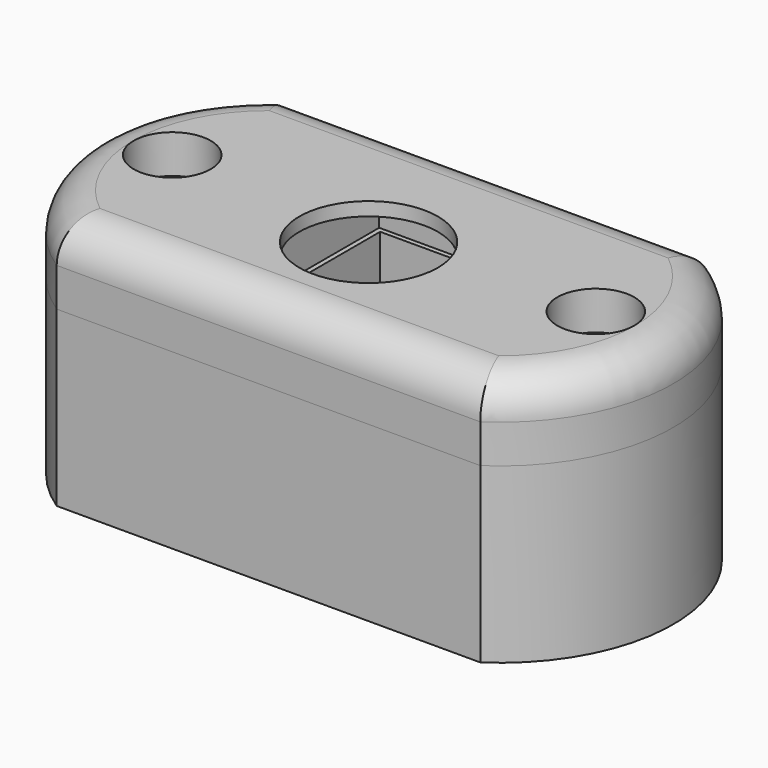
from build123d import *

# Parameters (mm, degrees)
F0_W            = 22
F0_H            = 15
F1_DEPTH        = 9
F2_R            = 1
F2_W            = 10
F2_H            = 12
F3_DEPTH        = 9
F4_W            = 10
F4_H            = 9
F5_DEPTH        = 0.5
F6_W            = 22
F6_H            = 15
F7_DEPTH        = 4
F8_R            = 3.6
F9_DEPTH        = 4
F10_T1_DEPTH    = 32
F10_T4_ANGLE    = 176.5875970816
F10_T6_ANGLE    = 176.5875970816
F11_D           = 2
F11_DEPTH       = 20
F11_CBORE_D     = 4
F11_CBORE_DEPTH = 2
F11_TIP         = 0.600860619
F12_W           = 10.5
F12_H           = 12.5
F13_DEPTH       = 3.3


# Not quite as in the source:
# - a fillet or chamfer that OpenCascade refuses, or shapes differently, is made with other operations: its cross-section is extruded or revolved along the edge and cut away or added


with BuildPart() as f1:
    # F0 (on Top) → F1 (new body)
    with BuildSketch(Plane.XY):
        with Locations((-45, -43.5413755476)):
            Rectangle(F0_W, F0_H)
        with BuildLine():
            ThreePointArc((-34, -51.0413755476), (-29.9749371855, -43.5413755476), (-34, -36.0413755476))
            Line((-34, -36.0413755476), (-34, -51.0413755476))
        make_face()
        with BuildLine():
            Line((-56, -51.0413755476), (-56, -36.0413755476))
            ThreePointArc((-56, -36.0413755476), (-60.0250628145, -43.5413755476), (-56, -51.0413755476))
        make_face()
    extrude(amount=F1_DEPTH)

    # F2 (on face) → F3 (cut)
    with BuildSketch(Plane.XY.offset(9)):
        with Locations((-56, -43.5413755476)):
            Circle(F2_R)
        with Locations((-34, -43.5413755476)):
            Circle(F2_R)
        with Locations((-45, -43.5413755476)):
            Rectangle(F2_W, F2_H)
    extrude(amount=-F3_DEPTH, mode=Mode.SUBTRACT)

    # F4 (on face) → F5 (join)
    with BuildSketch(Plane(origin=(0, 0, 0), x_dir=(1, 0, 0), z_dir=(0, 0, -1))):
        with Locations((-45, 45.0413755476)):
            Rectangle(F4_W, F4_H)
    extrude(amount=-F5_DEPTH)


with BuildPart() as f7:
    # F6 (on face) → F7 (new body)
    with BuildSketch(Plane.XY.offset(9)):
        with Locations((-45, -43.5413755476)):
            Rectangle(F6_W, F6_H)
        with BuildLine():
            ThreePointArc((-34, -51.0413755476), (-29.9749371855, -43.5413755476), (-34, -36.0413755476))
            Line((-34, -36.0413755476), (-34, -51.0413755476))
        make_face()
        with BuildLine():
            Line((-56, -51.0413755476), (-56, -36.0413755476))
            ThreePointArc((-56, -36.0413755476), (-60.0250628145, -43.5413755476), (-56, -51.0413755476))
        make_face()
    extrude(amount=F7_DEPTH)

    # F8 (on face) → F9 (cut)
    with BuildSketch(Plane.XY.offset(13)):
        with Locations((-45, -44.5413755476)):
            Circle(F8_R)
    extrude(amount=-F9_DEPTH, mode=Mode.SUBTRACT)

    # F10: fillet of radius 2 on 4 edges, made by hand

    # F10_s2 → F10_t1 (cut)
    with BuildSketch(Plane.YZ.offset(-61)):
        with BuildLine():
            ThreePointArc((-36.0413755476, 11), (-36.6271619853, 12.4142135624), (-38.0413755476, 13))
            Line((-38.0413755476, 13), (-36.0413755476, 13))
            Line((-36.0413755476, 13), (-36.0413755476, 11))
        make_face()
        with BuildLine():
            ThreePointArc((-49.0413755476, 13), (-50.45558911, 12.4142135624), (-51.0413755476, 11))
            Line((-51.0413755476, 11), (-51.0413755476, 13))
            Line((-51.0413755476, 13), (-49.0413755476, 13))
        make_face()
    extrude(amount=F10_T1_DEPTH, mode=Mode.SUBTRACT)

    # F10_s3 → F10_t4 (revolve, cut)
    with BuildSketch(Plane(origin=(-40.2362302043, -1.1985422881, 0), x_dir=(0, 0, 1), z_dir=(-0.9995566433, -0.0297744322, 0))):
        with BuildLine():
            ThreePointArc((11, -51.3616145647), (12.4142135624, -50.7758281271), (13, -49.3616145647))
            Line((13, -49.3616145647), (13, -51.3616145647))
            Line((13, -51.3616145647), (11, -51.3616145647))
        make_face()
    revolve(axis=Axis((-38.9749371855, -43.5413755476, 13), (0, 0, 1)), revolution_arc=F10_T4_ANGLE, mode=Mode.SUBTRACT)

    # F10_s5 → F10_t6 (revolve, cut)
    with BuildSketch(Plane(origin=(-52.2756731943, -1.557168866, 0), x_dir=(0, 0, 1), z_dir=(0.9995566433, 0.0297744322, 0))):
        with BuildLine():
            ThreePointArc((11, 33.0028289167), (12.4142135624, 33.5886153543), (13, 35.0028289167))
            Line((13, 35.0028289167), (13, 33.0028289167))
            Line((13, 33.0028289167), (11, 33.0028289167))
        make_face()
    revolve(axis=Axis((-51.0250628145, -43.5413755476, 13), (0, 0, 1)), revolution_arc=F10_T6_ANGLE, mode=Mode.SUBTRACT)

    # F11
    with Locations(Plane.XY.offset(13)):
        with Locations((-34, -43.5413755476), (-56, -43.5413755476)):
            CounterBoreHole(F11_D / 2, F11_CBORE_D / 2, F11_CBORE_DEPTH, depth=F11_DEPTH)
            with Locations((0, 0, -(F11_DEPTH + F11_TIP / 2))):  # 118° drill point
                Cone(0, F11_D / 2, F11_TIP, mode=Mode.SUBTRACT)

    # F12 (on face) → F13 (cut)
    with BuildSketch(Plane(origin=(0, 0, 9), x_dir=(1, 0, 0), z_dir=(0, 0, -1))):
        with Locations((-45, 43.5413755476)):
            Rectangle(F12_W, F12_H)
    extrude(amount=-F13_DEPTH, mode=Mode.SUBTRACT)


solid = Compound([f1.part, f7.part])
